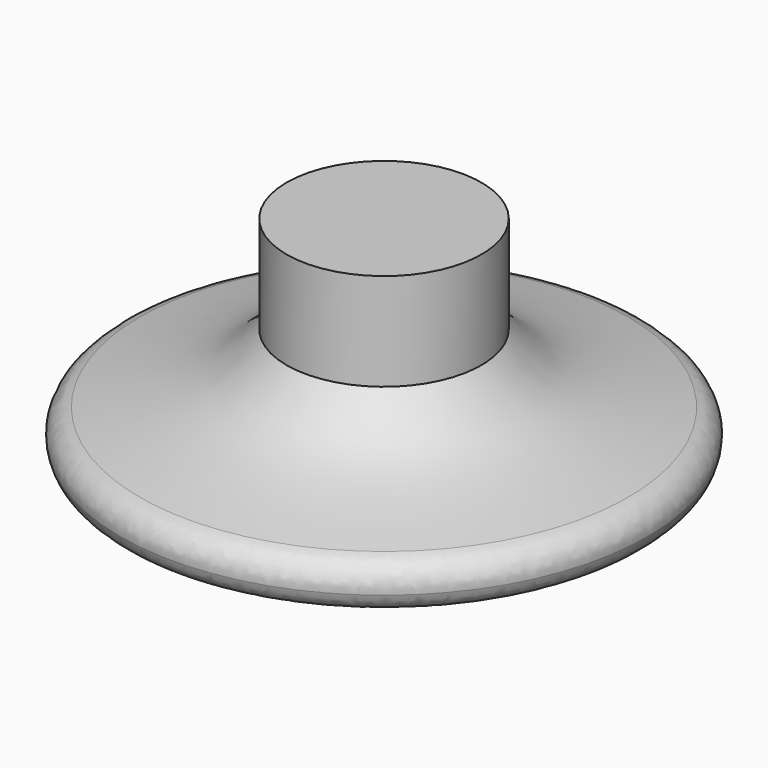
from build123d import *

# Parameters (mm, degrees)
F0_W = 4
F0_H = 4
F2_R = 0.99999


# Not quite as in the source:
# - a fillet or chamfer is up to 0.001 mm smaller than in the source, because OpenCascade refuses the exact size
# - the dataset's text gives a spline's control points without its knots; the knots are read off the source's solid


with BuildPart() as f1:
    # F0 (on Front) → F1 (revolve)
    with BuildSketch(Plane.XZ):
        with BuildLine():
            Line((0.9091711268, 3), (-3.0908288732, 3))
            add(Edge.make_bspline(
                [(-3.0908288732, 3), (-3.5834098611, 2.4200538723), (-4.8095609066, 0.976430248), (-8.1139250982, 0.3655009849), (-10.0908288732, 0)],
                knots=[0, 0, 0, 0, 0.4017294522, 1, 1, 1, 1], degree=3))
            Line((-10.0908288732, 0), (-9.7272200714, -1.9666694281))
            add(Edge.make_bspline(
                [(-1.5664662541, 1.7052727679), (-1.7197351348, 1.5248198149), (-2.063357916, 1.1180932901), (-2.6429158857, 0.5377987308), (-3.2231154482, 0.0813793664), (-3.7171330132, -0.2427740222), (-4.2708452388, -0.5352938299), (-4.8332722817, -0.7761481117), (-5.411616192, -0.9839057168), (-6.200976021, -1.2257159643), (-7.2204637167, -1.4786072566), (-8.4760577728, -1.735410051), (-9.3141745474, -1.8903032702), (-9.7272200714, -1.9666694281)],
                knots=[0, 0, 0, 0, 0.125, 0.25, 0.3125, 0.375, 0.4375, 0.5, 0.5625, 0.625, 0.75, 0.875, 1, 1, 1, 1], degree=3))
            Line((-1.5664662541, 1.7052727679), (0.9091711268, 3))
        make_face()
        with Locations((-1.0908288732, 5)):
            Rectangle(F0_W, F0_H)
    revolve(axis=Axis((0.9091711268, 0, 5), (0, 0, 1)))

    # F2 (radius 1 in the source; OpenCascade refuses exactly that, so slightly less here)
    f2_edges = [f1.edges().sort_by_distance(p)[0] for p in [
        (11.545562, 0, -1.966669),
        (11.909171, 0, 0),
    ]]
    fillet(f2_edges, radius=F2_R)


solid = f1.part
